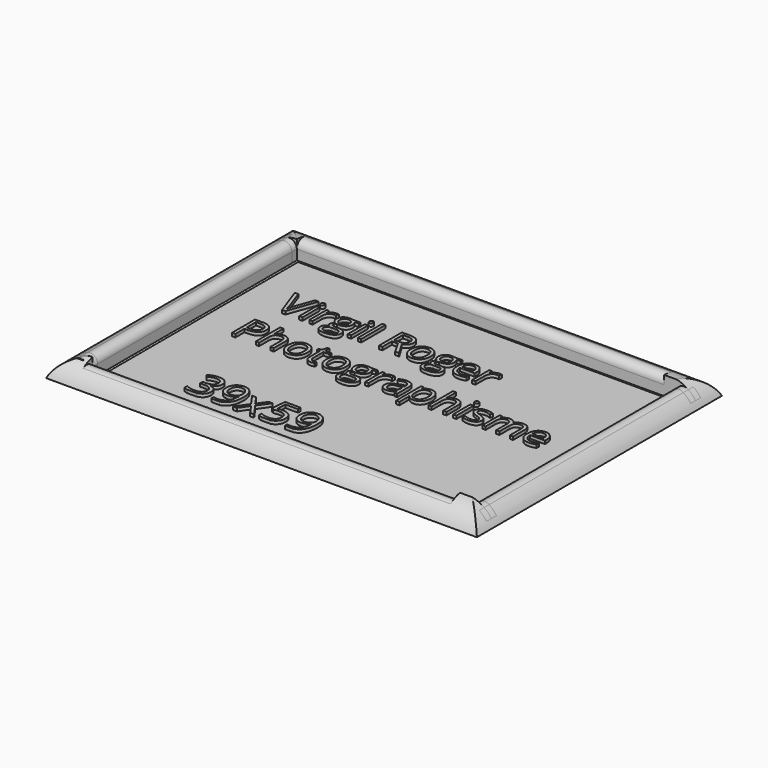
from build123d import *
from build123d import SkipClean  # not in build123d's __all__

# Parameters (mm, degrees)
F0_W           = 70
F0_H           = 50
F1_DEPTH       = 5
F2_W           = 1
F2_H           = 5
F2_H_2         = 1
F2_W_2         = 4
F2_H_3         = 39
F2_W_3         = 59
F2_H_4         = 4
F2_W_4         = 5
F3_DEPTH       = 2
F4_T           = 2.5
F4_T3_DEPTH    = 9
F4_T5_DEPTH    = 44
F4_T7_DEPTH    = 10
F4_T9_DEPTH    = 9
F4_T11_DEPTH   = 64
F4_T13_DEPTH   = 10
F5_TEXT_SIZE   = 6.4521332366
F5_TEXT_SIZE_2 = 7.0870937379
F6_DEPTH       = 0.5
F7_DEPTH       = 2.5
F8_T1_DEPTH    = 64
F8_T3_DEPTH    = 83.4948974279
F8_T5_DEPTH    = 63.4948974279
F8_T7_DEPTH    = 84
F9_DEPTH       = 1
F10_R          = 1.2
F11_DEPTH      = 2
F12_DEPTH      = 2
F13_DEPTH      = 2
F14_DEPTH      = 2


# Not quite as in the source:
# - a fillet or chamfer that OpenCascade refuses, or shapes differently, is made with other operations: its cross-section is extruded or revolved along the edge and cut away or added
# - after a boolean that leaves OpenCascade's solid faulty, fix() repairs it
# - a shell that OpenCascade refuses in one call is made with other operations: the cavity is built on its own and cut out
# - Text() gives the source's letters only with a copy of the font that has no kerning and outlines rounded to 1/6400 em; it was checked with that copy


with BuildPart() as f1:
    # F0 (on Top) → F1 (new body)
    with BuildSketch(Plane.XY):
        with Locations((3.4472942352, 8.8653620177)):
            Rectangle(F0_W, F0_H)
    extrude(amount=F1_DEPTH)

    # F2 (on face) → F3 (cut)
    with BuildSketch(Plane.XY.offset(5)):
        with Locations((33.9472942352, 31.3653620177)):
            Rectangle(F2_W, F2_H)
        with Locations((33.9472942352, 28.3653620177)):
            Rectangle(F2_W, F2_H_2)
        with Locations((36.4472942352, 28.3653620177)):
            Rectangle(F2_W_2, F2_H_2)
        with Locations((33.9472942352, 8.3653620177)):
            Rectangle(F2_W, F2_H_3)
        with Locations((3.9472942352, 28.3653620177)):
            Rectangle(F2_W_3, F2_H_2)
        with Locations((3.9472942352, -11.6346379823)):
            Rectangle(F2_W_3, F2_H_2)
        with Locations((36.4472942352, -11.6346379823)):
            Rectangle(F2_W_2, F2_H_2)
        with Locations((33.9472942352, -11.6346379823)):
            Rectangle(F2_W, F2_H_2)
        with Locations((33.9472942352, -14.1346379823)):
            Rectangle(F2_W, F2_H_4)
        with Locations((-26.0527057648, 31.3653620177)):
            Rectangle(F2_W, F2_H)
        with Locations((-26.0527057648, 28.3653620177)):
            Rectangle(F2_W, F2_H_2)
        with Locations((-29.0527057648, 28.3653620177)):
            Rectangle(F2_W_4, F2_H_2)
        with Locations((-26.0527057648, 8.3653620177)):
            Rectangle(F2_W, F2_H_3)
        with Locations((-26.0527057648, -11.6346379823)):
            Rectangle(F2_W, F2_H_2)
        with Locations((-29.0527057648, -11.6346379823)):
            Rectangle(F2_W_4, F2_H_2)
        with Locations((-26.0527057648, -14.1346379823)):
            Rectangle(F2_W, F2_H_4)
    extrude(amount=-F3_DEPTH, mode=Mode.SUBTRACT)

    # F4: shell of thickness 2.5, made by hand


with BuildPart() as f4_core1:
    # F4_t2: copy of F1
    add(f1.part, clean=False)

    # the walls: a layer under each face that stays
    f4_faces = [f4_core1.faces().sort_by_distance(p)[0] for p in [
        (38.4472942352, 8.8653620177, 2.5),
        (3.4472942352, 8.8653620177, 0),
        (3.4472942352, 33.8653620177, 2.5),
        (36.4472942352, 31.3653620177, 5),
        (36.4472942352, 28.8653620177, 4),
        (-27.1777057648, 28.3098064622, 3),
        (36.4472942352, 27.8653620177, 4),
        (36.4472942352, 8.3653620177, 5),
        (36.4472942352, -11.1346379823, 4),
        (36.4472942352, -12.1346379823, 4),
        (36.4472942352, -14.1346379823, 5),
        (3.4472942352, -16.1346379823, 2.5),
        (-31.5527057648, 8.8653620177, 2.5),
        (-29.0527057648, 31.3653620177, 5),
        (-26.5527057648, 31.3653620177, 4),
        (-25.5527057648, 31.3653620177, 4),
        (3.9472942352, 31.3653620177, 5),
        (33.4472942352, 31.3653620177, 4),
        (34.4472942352, 31.3653620177, 4),
        (-26.5527057648, 8.3653620177, 4),
        (-29.0527057648, -11.1346379823, 4),
        (-29.0527057648, -12.1346379823, 4),
        (-26.5527057648, -14.1346379823, 4),
        (-25.5527057648, -14.1346379823, 4),
        (3.9472942352, -12.1346379823, 4),
        (33.4472942352, -14.1346379823, 4),
        (34.4472942352, -14.1346379823, 4),
        (34.4472942352, 8.3653620177, 4),
        (3.9472942352, 28.8653620177, 4),
        (-29.0527057648, 28.8653620177, 4),
        (-29.0527057648, 27.8653620177, 4),
        (3.9472942352, -11.1346379823, 4),
        (-25.5527057648, 8.3653620177, 4),
        (3.9472942352, 27.8653620177, 4),
        (33.4472942352, 8.3653620177, 4),
        (3.9472942352, -14.1346379823, 5),
        (-29.0527057648, -14.1346379823, 5),
        (-29.0527057648, 8.3653620177, 5),
    ]]
    thicken(f4_faces, amount=-F4_T, mode=Mode.SUBTRACT)

    # F4_s4 → F4_t3 (cut)
    with BuildSketch(Plane.YZ.offset(31.9472942352)):
        Polygon((28.8403620177, 3.025), (31.3653620177, 3), (31.3653620177, 0.5), (28.8653620177, 0.5), align=None)
        Polygon((-12.1096379823, 3.025), (-12.1346379823, 0.5), (-14.6346379823, 0.5), (-14.6346379823, 3), align=None)
        Polygon((-11.1596379823, 3.025), (-11.1346379823, 0.5), (-8.6346379823, 0.5), (-8.6346379823, 3), align=None)
        Polygon((27.8903620177, 3.025), (27.8653620177, 0.5), (25.3653620177, 0.5), (25.3653620177, 3), align=None)
    extrude(amount=F4_T3_DEPTH, mode=Mode.SUBTRACT)

    # F4_s6 → F4_t5 (cut)
    with BuildSketch(Plane.XZ.offset(-30.3653620177)):
        Polygon((-26.5277057648, 3.025), (-26.5527057648, 0.5), (-29.0527057648, 0.5), (-29.0527057648, 3), align=None)
        Polygon((34.4222942352, 3.025), (34.4472942352, 0.5), (36.9472942352, 0.5), (36.9472942352, 3), align=None)
        Polygon((-25.5777057648, 3.025), (-25.5527057648, 0.5), (-23.0527057648, 0.5), (-23.0527057648, 3), align=None)
        Polygon((33.4722942352, 3.025), (33.4472942352, 0.5), (30.9472942352, 0.5), (30.9472942352, 3), align=None)
    extrude(amount=F4_T5_DEPTH, mode=Mode.SUBTRACT)

    # F4_s8 → F4_t7 (cut)
    with BuildSketch(Plane.YZ.offset(-34.0527057648)):
        Polygon((-11.1596379823, 3.025), (-11.1346379823, 0.5), (-8.6346379823, 0.5), (-8.6346379823, 3), align=None)
        Polygon((-12.1096379823, 3.025), (-12.1346379823, 0.5), (-14.6346379823, 0.5), (-14.6346379823, 3), align=None)
        Polygon((28.8403620177, 3.025), (28.8653620177, 0.5), (31.3653620177, 0.5), (31.3653620177, 3), align=None)
        Polygon((27.8903620177, 3.025), (27.8653620177, 0.5), (25.3653620177, 0.5), (25.3653620177, 3), align=None)
    extrude(amount=F4_T7_DEPTH, mode=Mode.SUBTRACT)

    # F4_s10 → F4_t9 (cut)
    with BuildSketch(Plane.XZ.offset(9.6346379823)):
        Polygon((-26.5277057648, 3.025), (-26.5527057648, 0.5), (-29.0527057648, 0.5), (-29.0527057648, 3), align=None)
        Polygon((-25.5777057648, 3.025), (-25.5527057648, 0.5), (-23.0527057648, 0.5), (-23.0527057648, 3), align=None)
        Polygon((33.4722942352, 3.025), (33.4472942352, 0.5), (30.9472942352, 0.5), (30.9472942352, 3), align=None)
        Polygon((34.4222942352, 3.025), (34.4472942352, 0.5), (36.9472942352, 0.5), (36.9472942352, 3), align=None)
    extrude(amount=F4_T9_DEPTH, mode=Mode.SUBTRACT)

    # F4_s12 → F4_t11 (cut)
    with BuildSketch(Plane.YZ.offset(-28.0527057648)):
        Polygon((-12.1096379823, 3.025), (-12.1346379823, 0.5), (-14.6346379823, 0.5), (-14.6346379823, 3), align=None)
        Polygon((28.8403620177, 3.025), (28.8653620177, 0.5), (31.3653620177, 0.5), (31.3653620177, 3), align=None)
        Polygon((-11.1596379823, 3.025), (-11.1346379823, 0.5), (-8.6346379823, 0.5), (-8.6346379823, 3), align=None)
        Polygon((27.8903620177, 3.025), (27.8653620177, 0.5), (25.3653620177, 0.5), (25.3653620177, 3), align=None)
    extrude(amount=F4_T11_DEPTH, mode=Mode.SUBTRACT)

    # F4_s14 → F4_t13 (cut)
    with BuildSketch(Plane.XZ.offset(-36.3653620177)):
        Polygon((34.4222942352, 3.025), (34.4472942352, 0.5), (36.9472942352, 0.5), (36.9472942352, 3), align=None)
        Polygon((33.4722942352, 3.025), (33.4472942352, 0.5), (30.9472942352, 0.5), (30.9472942352, 3), align=None)
        Polygon((-25.5777057648, 3.025), (-25.5527057648, 0.5), (-23.0527057648, 0.5), (-23.0527057648, 3), align=None)
        Polygon((-26.5277057648, 3.025), (-26.5527057648, 0.5), (-29.0527057648, 0.5), (-29.0527057648, 3), align=None)
    extrude(amount=F4_T13_DEPTH, mode=Mode.SUBTRACT)


with BuildPart() as f1_1:
    add(f1.part, clean=False)

    # what is left inside the walls is the cavity
    f4_cavity = [f4_core1.part.solids().sort_by_distance(p)[0] for p in [
        (3.947294, 2.698695, 4.975),
    ]]
    add(f4_cavity, mode=Mode.SUBTRACT)

    # F5 (on face) → F6 (join)
    with BuildSketch(Plane.XY.offset(2.5)):
        with Locations((-20.0527057648, 15.7198260874)):
            Text('Virgil Roger', F5_TEXT_SIZE, font='Open Sans', text_align=(TextAlign.LEFT, TextAlign.BOTTOM))
        with Locations((-20.0527057648, 6.9449248857)):
            Text('Photographisme', F5_TEXT_SIZE, font='Open Sans', text_align=(TextAlign.LEFT, TextAlign.BOTTOM))
        with Locations((-15.0800719857, -8.6346379823)):
            Text('39x59', F5_TEXT_SIZE_2, font='Open Sans', text_align=(TextAlign.LEFT, TextAlign.BOTTOM))
    extrude(amount=F6_DEPTH)

    # F7 (cut): a face of the model
    f7_faces = [f1_1.faces().sort_by_distance(p)[0] for p in [
        (3.9472942352, -10.4273897939, 5),
    ]]
    extrude(f7_faces, amount=-F7_DEPTH, mode=Mode.SUBTRACT)

    # F8: fillet of radius 5 on 4 edges, made by hand

    # F8_s2 → F8_t1 (cut)
    with BuildSketch(Plane.XZ.offset(-40.3653620177)):
        with BuildLine():
            ThreePointArc((-31.5527057648, 0), (-30.0882396707, 3.5355339059), (-26.5527057648, 5))
            Line((-26.5527057648, 5), (-31.5527057648, 5))
            Line((-31.5527057648, 5), (-31.5527057648, 0))
        make_face()
    extrude(amount=F8_T1_DEPTH, mode=Mode.SUBTRACT)

    # F8_s4 → F8_t3 (cut)
    with BuildSketch(Plane.YZ.offset(-37.8001544787)):
        with BuildLine():
            ThreePointArc((-16.1346379823, 0.1010205144), (-15.0076213285, 3.2632981746), (-12.1346379823, 5))
            Line((-12.1346379823, 5), (-16.1346379823, 5))
            Line((-16.1346379823, 5), (-16.1346379823, 0.1010205144))
        make_face()
    extrude(amount=F8_T3_DEPTH, mode=Mode.SUBTRACT)

    # F8_s6 → F8_t5 (cut)
    with BuildSketch(Plane.XZ.offset(-40.1128107317)):
        with BuildLine():
            ThreePointArc((38.4472942352, 0.1010205144), (37.3202775814, 3.2632981746), (34.4472942352, 5))
            Line((34.4472942352, 5), (38.4472942352, 5))
            Line((38.4472942352, 5), (38.4472942352, 0.1010205144))
        make_face()
    extrude(amount=F8_T5_DEPTH, mode=Mode.SUBTRACT)

    # F8_s8 → F8_t7 (cut)
    with BuildSketch(Plane.YZ.offset(-38.0527057648)):
        with BuildLine():
            ThreePointArc((33.8653620177, 0), (32.4008959237, 3.5355339059), (28.8653620177, 5))
            Line((28.8653620177, 5), (33.8653620177, 5))
            Line((33.8653620177, 5), (33.8653620177, 0))
        make_face()
    extrude(amount=F8_T7_DEPTH, mode=Mode.SUBTRACT)

    # F9 (cut): a face of the model
    f9_faces = [f1_1.faces().sort_by_distance(p)[0] for p in [
        (-29.7193310272, 28.3653620177, 3),
    ]]
    extrude(f9_faces, amount=-F9_DEPTH, mode=Mode.SUBTRACT)

    # F10
    f10_edges = [f1_1.edges().sort_by_distance(p)[0] for p in [
        (3.947294, -12.134638, 5),
        (-26.552706, 8.365362, 5),
        (34.447294, 8.365362, 5),
        (3.947294, 28.865362, 5),
    ]]
    fillet(f10_edges, radius=F10_R)

    # F11 (cut): a face of the model
    f11_faces = [f1_1.faces().sort_by_distance(p)[0] for p in [
        (3.4472942352, 8.8653620177, 0),
    ]]
    extrude(f11_faces, amount=-F11_DEPTH, mode=Mode.SUBTRACT)

    # F12 (add): faces of the model
    f12_faces = [f1_1.faces().sort_by_distance(p)[0] for p in [
        (-25.5527057648, -13.5764726132, 3.0363271791),
        (-25.5527057648, 30.6771011935, 3.1915273358),
        (34.4472942352, 30.6030677952, 3.2668868616),
        (34.4472942352, -13.4560876061, 3.2099140304),
    ]]
    extrude(f12_faces, amount=F12_DEPTH)

    # F13 (add): faces of the model
    f13_faces = [f1_1.faces().sort_by_distance(p)[0] for p in [
        (-28.3644449405, -11.1346379823, 3.1915273358),
        (35.8891288661, -11.1346379823, 3.0363271791),
    ]]
    with SkipClean():  # cleaning this boolean's faces spoils the solid; the shape is the same uncleaned
        extrude(f13_faces, amount=F13_DEPTH)

    # F14 (add): faces of the model
    f14_faces = [f1_1.faces().sort_by_distance(p)[0] for p in [
        (35.8891288661, 27.8653620177, 3.0363271791),
        (-28.3644449405, 27.8653620177, 3.1915273358),
    ]]
    extrude(f14_faces, amount=F14_DEPTH)

    add(f1_1.part.fix(), mode=Mode.REPLACE)


solid = f1_1.part
